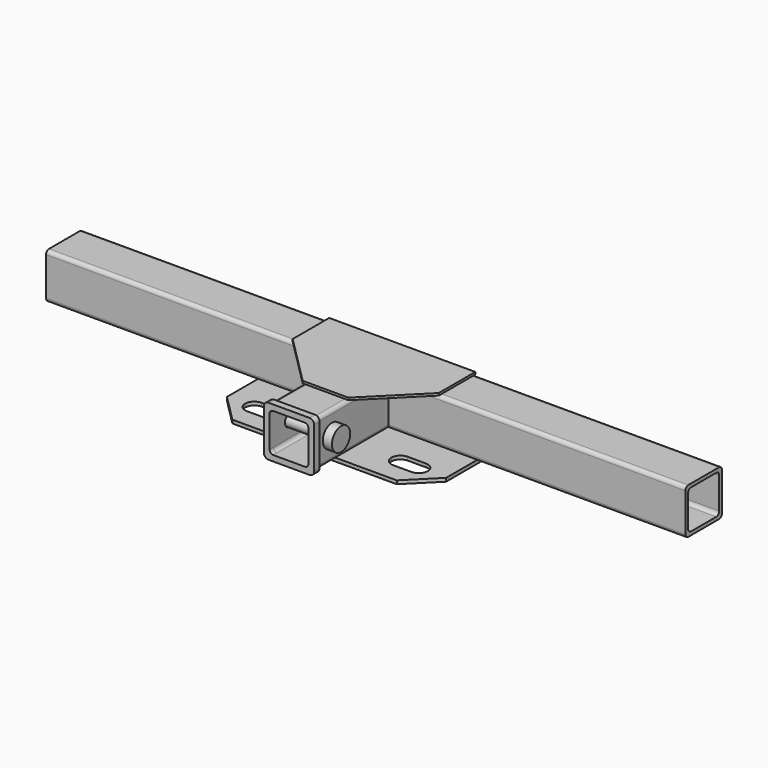
from build123d import *

# Parameters (mm, degrees)
F0_W           = 63.5
F0_H           = 63.5
F0_W_2         = 53.975
F0_H_2         = 53.975
F1_DEPTH       = 444.5
F2_W           = 63.5
F2_H           = 63.5
F2_W_2         = 53.975
F2_H_2         = 53.975
F3_DEPTH       = 127
F3_DEPTH_BACK  = 63.5
F4_R           = 5.08
F6_DEPTH       = 3.175
F8_DEPTH       = 4.7625
F10_DEPTH      = 6.35
F10_DEPTH_BACK = 3.175
F12_R          = 8.3312
F13_DEPTH      = 476.251
F14_R          = 15.875
F15_DEPTH      = 12.7
F16_R          = 7.9375
F17_DEPTH      = 76.2


with BuildPart() as f1:
    # F0 (on Right) → F1 (new body, symmetric)
    with BuildSketch(Plane.YZ):
        with Locations((-58.7375, -31.75)):
            Rectangle(F0_W, F0_H)
        with Locations((-58.7375, -31.75)):
            Rectangle(F0_W_2, F0_H_2, mode=Mode.SUBTRACT)
    extrude(amount=F1_DEPTH, both=True)

    # F2 (on face) → F3 (join, two sides)
    with BuildSketch(Plane.XZ.offset(90.4875)) as f3_sk:
        with Locations((0, -31.75)):
            Rectangle(F2_W, F2_H)
        with Locations((0, -31.75)):
            Rectangle(F2_W_2, F2_H_2, mode=Mode.SUBTRACT)
    extrude(amount=F3_DEPTH)
    extrude(f3_sk.sketch, amount=-F3_DEPTH_BACK)

    # F4
    f4_edges = [f1.edges().sort_by_distance(p)[0] for p in [
        (-238.125, -90.4875, 0),
        (238.125, -90.4875, 0),
        (0, -26.9875, 0),
        (0, -26.9875, -63.5),
        (-238.125, -90.4875, -63.5),
        (238.125, -90.4875, -63.5),
        (0, -31.75, -4.7625),
        (0, -85.725, -4.7625),
        (0, -31.75, -58.7375),
        (0, -85.725, -58.7375),
        (-31.75, -153.9875, 0),
        (31.75, -153.9875, 0),
        (31.75, -153.9875, -63.5),
        (-31.75, -153.9875, -63.5),
        (-26.9875, -153.9875, -4.7625),
        (26.9875, -153.9875, -4.7625),
        (-26.9875, -153.9875, -58.7375),
        (26.9875, -153.9875, -58.7375),
        (238.125, -85.725, -58.7375),
        (238.125, -85.725, -4.7625),
        (238.125, -31.75, -58.7375),
        (238.125, -31.75, -4.7625),
        (-238.125, -85.725, -4.7625),
        (-238.125, -85.725, -58.7375),
        (-238.125, -31.75, -58.7375),
        (-238.125, -31.75, -4.7625),
    ]]
    fillet(f4_edges, radius=F4_R)

    # F5 (on face) → F6 (join)
    with BuildSketch(Plane.XY):
        Polygon((101.6, -26.9875), (-101.6, -26.9875), (-101.6, -90.4875), (-31.75, -90.4875), (-31.75, -160.3375), (31.75, -160.3375), (31.75, -90.4875), (101.6, -90.4875), align=None)
        Polygon((-31.75, -90.4875), (-101.6, -90.4875), (-31.75, -160.3375), align=None)
        Polygon((31.75, -160.3375), (101.6, -90.4875), (31.75, -90.4875), align=None)
    extrude(amount=F6_DEPTH)

    # F7 (on face) → F8 (join)
    with BuildSketch(Plane(origin=(0, 0, -63.5), x_dir=(1, 0, 0), z_dir=(0, 0, -1))):
        Polygon((-152.4, 26.9875), (152.4, 26.9875), (152.4, 141.2875), (114.3, 179.3875), (-114.3, 179.3875), (-152.4, 141.2875), align=None)
        with BuildLine():
            ThreePointArc((-127, 141.2875), (-123.2802561211, 150.2677561211), (-114.3, 153.9875))
            Line((-114.3, 153.9875), (-88.9, 153.9875))
            ThreePointArc((-88.9, 153.9875), (-79.9197438789, 150.2677561211), (-76.2, 141.2875))
            ThreePointArc((-76.2, 141.2875), (-79.9197438789, 132.3072438789), (-88.9, 128.5875))
            Line((-88.9, 128.5875), (-114.3, 128.5875))
            ThreePointArc((-114.3, 128.5875), (-123.2802561211, 132.3072438789), (-127, 141.2875))
        make_face(mode=Mode.SUBTRACT)
        with BuildLine():
            Line((114.3, 128.5875), (88.9, 128.5875))
            ThreePointArc((88.9, 128.5875), (79.9197438789, 132.3072438789), (76.2, 141.2875))
            ThreePointArc((76.2, 141.2875), (79.9197438789, 150.2677561211), (88.9, 153.9875))
            Line((88.9, 153.9875), (114.3, 153.9875))
            ThreePointArc((114.3, 153.9875), (123.2802561211, 150.2677561211), (127, 141.2875))
            ThreePointArc((127, 141.2875), (123.2802561211, 132.3072438789), (114.3, 128.5875))
        make_face(mode=Mode.SUBTRACT)
    extrude(amount=F8_DEPTH)

    # F9 (on face) → F10 (join, two sides)
    with BuildSketch(Plane.XZ.offset(217.4875)) as f10_sk:
        with BuildLine():
            Line((28.575, 3.175), (-28.575, 3.175))
            ThreePointArc((-28.575, 3.175), (-33.0651280605, 1.3151280605), (-34.925, -3.175))
            Line((-34.925, -3.175), (-34.925, -60.325))
            ThreePointArc((-34.925, -60.325), (-33.0651280605, -64.8151280605), (-28.575, -66.675))
            Line((-28.575, -66.675), (28.575, -66.675))
            ThreePointArc((28.575, -66.675), (33.0651280605, -64.8151280605), (34.925, -60.325))
            Line((34.925, -60.325), (34.925, -3.175))
            ThreePointArc((34.925, -3.175), (33.0651280605, 1.3151280605), (28.575, 3.175))
        make_face()
        with BuildLine():
            ThreePointArc((-26.9875, -9.8425), (-25.4996024484, -6.2503975516), (-21.9075, -4.7625))
            Line((-21.9075, -4.7625), (21.9075, -4.7625))
            ThreePointArc((21.9075, -4.7625), (25.4996024484, -6.2503975516), (26.9875, -9.8425))
            Line((26.9875, -9.8425), (26.9875, -53.6575))
            ThreePointArc((26.9875, -53.6575), (25.4996024484, -57.2496024484), (21.9075, -58.7375))
            Line((21.9075, -58.7375), (-21.9075, -58.7375))
            ThreePointArc((-21.9075, -58.7375), (-25.4996024484, -57.2496024484), (-26.9875, -53.6575))
            Line((-26.9875, -53.6575), (-26.9875, -9.8425))
        make_face(mode=Mode.SUBTRACT)
    extrude(amount=F10_DEPTH)
    extrude(f10_sk.sketch, amount=-F10_DEPTH_BACK)

    # F12 (on face) → F13 (cut, through all)
    with BuildSketch(Plane.YZ.offset(31.75)):
        with Locations((-188.9125, -31.75)):
            Circle(F12_R)
    extrude(amount=-F13_DEPTH, mode=Mode.SUBTRACT)


with BuildPart() as f15:
    # F14 (on face) → F15 (new body)
    with BuildSketch(Plane.YZ.offset(31.75)):
        with Locations((-188.9125, -31.75)):
            Circle(F14_R)
    extrude(amount=F15_DEPTH)

    # F16 (on face) → F17 (join)
    with BuildSketch(Plane(origin=(31.75, 0, 0), x_dir=(0, -1, 0), z_dir=(-1, 0, 0))):
        with Locations((188.9125, -31.75)):
            Circle(F16_R)
    extrude(amount=F17_DEPTH)


solid = Compound([f1.part, f15.part])
